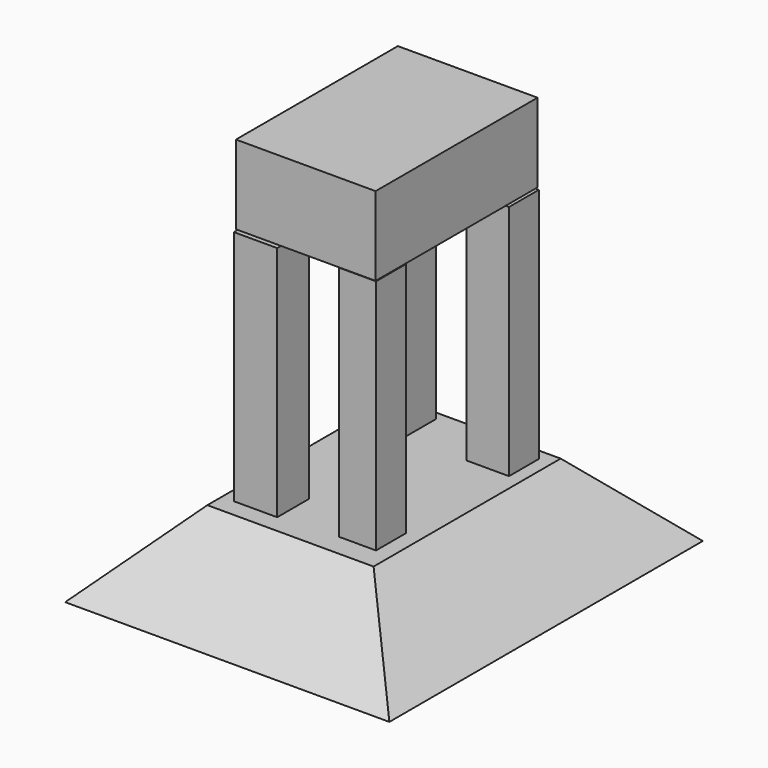
from build123d import *

# Parameters (mm, degrees)
F0_W     = 104.2639054358
F0_H     = 126.0087862611
F1_DEPTH = 25.4
F2_SIZE  = 25.39999
F3_W     = 12.2663415968
F3_H     = 14.2178032547
F3_W_2   = 13.6602446437
F3_H_2   = 11.9875594974
F3_W_3   = 13.9390230179
F3_H_3   = 12.8239002079
F3_W_4   = 11.9875576347
F3_H_4   = 11.9875632226
F4_DEPTH = 76.2
F5_W     = 44.9166167527
F5_H     = 65.0939904153
F6_DEPTH = 25.4


# Not quite as in the source:
# - a fillet or chamfer is up to 0.001 mm smaller than in the source, because OpenCascade refuses the exact size


with BuildPart() as f1:
    # F0 (on Top) → F1 (new body)
    with BuildSketch(Plane.XY):
        with Locations((4.5998785645, -1.3939030468)):
            Rectangle(F0_W, F0_H)
    extrude(amount=F1_DEPTH)

    # F2 (size 25.4 in the source; OpenCascade refuses exactly that, so slightly less here)
    f2_edges = [f1.edges().sort_by_distance(p)[0] for p in [
        (-47.532074, -1.393903, 25.4),
        (4.599879, -64.398296, 25.4),
        (56.731831, -1.393903, 25.4),
        (4.599879, 61.61049, 25.4),
    ]]
    chamfer(f2_edges, length=F2_SIZE)

    # F3 (on face) → F4 (join)
    with BuildSketch(Plane.XY.offset(25.4)):
        with Locations((-12.6845128834, 26.3447565958)):
            Rectangle(F3_W, F3_H)
        with Locations((20.3509759158, 26.6235359013)):
            Rectangle(F3_W_2, F3_H_2)
        with Locations((-11.2906098366, -26.7629260197)):
            Rectangle(F3_W_3, F3_H_3)
        with Locations((20.3509749845, -25.7871951908)):
            Rectangle(F3_W_4, F3_H_4)
    extrude(amount=F4_DEPTH)

    # F5 (on face) → F6 (join)
    with BuildSketch(Plane.XY.offset(101.6)):
        with Locations((3.6406246945, 0.9066630155)):
            Rectangle(F5_W, F5_H)
    extrude(amount=F6_DEPTH)


solid = f1.part
